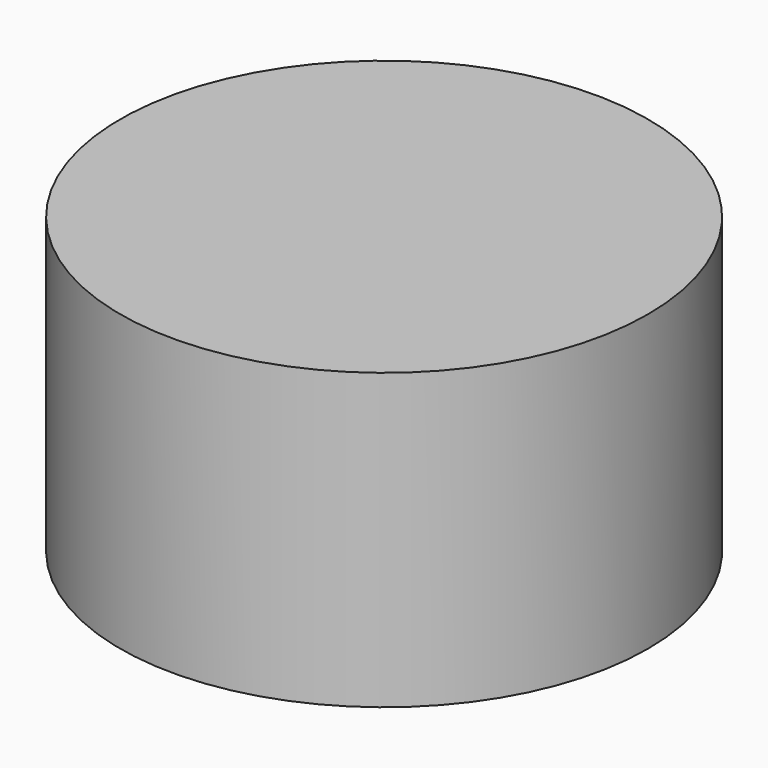
from build123d import *

# Parameters (mm, degrees)
F2_R     = 22.4134613052
F3_DEPTH = 25


# Not quite as in the source:
# - the program builds the solid bodies; features that only make, move or delete a surface that nothing else refers to are left out


with BuildPart() as f3:
    # F2 (on Top) → F3 (new body)
    with BuildSketch(Plane.XY):
        Circle(F2_R)
    extrude(amount=F3_DEPTH)


solid = f3.part
